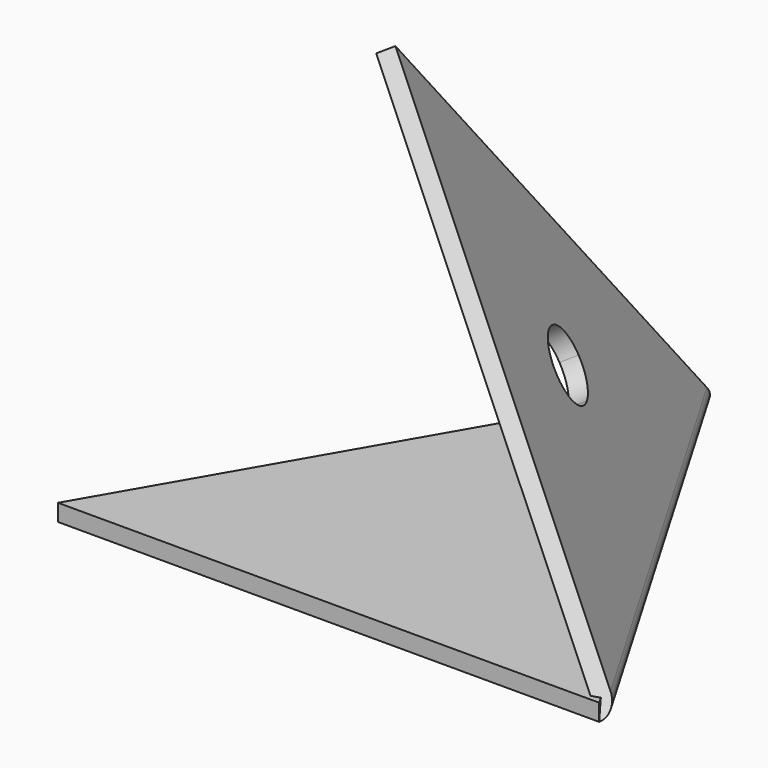
from build123d import *

# Parameters (mm, degrees)
F1_DEPTH    = 3.175
F5_DEPTH    = 3.175
F6_T1_DEPTH = 117.475
F8_DEPTH    = 3.175


# Not quite as in the source:
# - a fillet or chamfer that OpenCascade refuses, or shapes differently, is made with other operations: its cross-section is extruded or revolved along the edge and cut away or added


with BuildPart() as f1:
    # F0 (on Top) → F1 (new body)
    with BuildSketch(Plane.XY):
        Polygon((50.8, 0), (0, 87.9881810245), (-50.8, 0), align=None)
    extrude(amount=F1_DEPTH)

    # F4 (on line) → F5 (join)
    with BuildSketch(Plane(origin=(30.2473107364, 17.7959839325, 17.4632910558), x_dir=(-0.3931673168, 0.8910065242, -0.226995231), z_dir=(0.7716343063, 0.4539904997, 0.445503225))):
        Polygon((6.5029600393, 75.2459340132), (-19.9755570322, -25.4006840255), (78.3980433443, 0), align=None)
    extrude(amount=F5_DEPTH)

    # F6: fillet of radius 3.175 on 1 edges, made by hand

    # F6_s2 → F6_t1 (cut)
    with BuildSketch(Plane(origin=(17.005719551, -29.012184774, 0.1101218851), x_dir=(-0.862716434, -0.5056880012, 0), z_dir=(-0.5056852899, 0.8627118085, -0.0032746052))):
        with BuildLine():
            ThreePointArc((-45.25402581, 4.1728704395), (-45.421662158, 1.7486197382), (-43.8259948462, -0.0841211704))
            Line((-43.8259948462, -0.0841211704), (-46.668506133, 1.3303591527))
            Line((-46.668506133, 1.3303591527), (-45.25402581, 4.1728704395))
        make_face()
    extrude(amount=F6_T1_DEPTH, mode=Mode.SUBTRACT)

    # F7 (on face) → F8 (cut, through all)
    with BuildSketch(Plane(origin=(32.697249659, 19.2374037692, 18.877763795), x_dir=(-0.3931673168, 0.8910065242, -0.226995231), z_dir=(0.7716343063, 0.4539904997, 0.445503225))):
        with BuildLine():
            ThreePointArc((23.2165575735, 13.9849704437), (26.5917627129, 16.2568894847), (27.8951978201, 20.1110668007))
            ThreePointArc((27.8951978201, 20.1110668007), (25.399375136, 25.1576316934), (19.8738380667, 26.2371631576))
            Line((19.8738380667, 26.2371631576), (23.2165575735, 13.9849704437))
        make_face()
        with BuildLine():
            Line((23.2165575735, 13.9849704437), (19.8738380667, 26.2371631576))
            ThreePointArc((19.8738380667, 26.2371631576), (15.4191014631, 18.4397070472), (23.2165575735, 13.9849704437))
        make_face()
    extrude(amount=-F8_DEPTH, mode=Mode.SUBTRACT)


solid = f1.part
